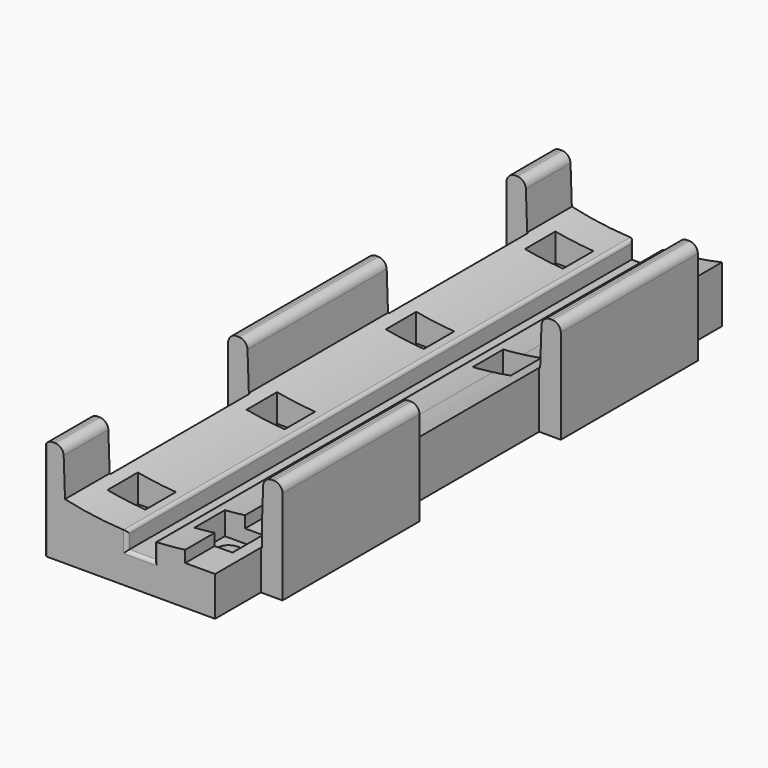
from build123d import *

# Parameters (mm, degrees)
F1_DEPTH     = 185
F3_DEPTH     = 30
F2_W         = 6.328
F2_H         = 51.6
F2_H_2       = 16.7
F2_H_3       = 50.8
F4_DEPTH     = 30
F5_D         = 6.7564
F6_START     = -7.6
F2_W_2       = 5.5565
F2_H_4       = 5.5565
F6_DEPTH     = 22.401
F7_T1_DEPTH  = 8
F7_T3_DEPTH  = 7.5701702527
F7_T5_DEPTH  = 35
F7_T7_DEPTH  = 189.78118177
F7_T13_DEPTH = 10.5
F7_T17_DEPTH = 10.0701702527
F7_T24_DEPTH = 10.0701702527
F7_T28_DEPTH = 10.5
F7_T35_DEPTH = 10.5
F7_T39_DEPTH = 10.0701702527
F7_T46_DEPTH = 10.0701702527
F7_T50_DEPTH = 10.5
F8_T1_DEPTH  = 27.8
F8_T3_DEPTH  = 28.3686226101
F8_T5_DEPTH  = 62.8686226101
F8_T7_DEPTH  = 63.3
F8_T9_DEPTH  = 27.8
F8_T11_DEPTH = 28.3686226101
F8_T13_DEPTH = 62.0686226101
F8_T15_DEPTH = 62.5
F8_T17_DEPTH = 62.5
F8_T19_DEPTH = 62.0686226101


# Not quite as in the source:
# - a fillet or chamfer that OpenCascade refuses, or shapes differently, is made with other operations: its cross-section is extruded or revolved along the edge and cut away or added
# - a feature names something its author has since deleted; it is built from what else it names


with BuildPart() as f1:
    # F0 (on Front) → F1 (new body)
    with BuildSketch(Plane.XZ):
        with BuildLine():
            Line((-28.0998, -84.153), (-28.0998, -96.0750292217))
            ThreePointArc((-28.0998, -96.0750292217), (-25.0871251247, -96.9053463591), (-22.05, -97.6412182431))
            Line((-22.05, -97.6412182431), (-22.5238, -84.153))
            Line((-22.5238, -84.153), (-28.0998, -84.153))
        make_face()
        with BuildLine():
            ThreePointArc((22.05, -97.6412182431), (25.0871251247, -96.9053463591), (28.0998, -96.0750292217))
            Line((28.0998, -96.0750292217), (28.0998, -84.153))
            Line((28.0998, -84.153), (22.5238, -84.153))
            Line((22.5238, -84.153), (22.05, -97.6412182431))
        make_face()
        with BuildLine():
            Line((22.05, -102.6412182431), (22.05, -97.6412182431))
            ThreePointArc((22.05, -97.6412182431), (17.5683261722, -98.5462526711), (13.05, -99.2456926017))
            Line((13.05, -99.2456926017), (13.05, -102.6412182431))
            Line((13.05, -102.6412182431), (22.05, -102.6412182431))
        make_face()
        with BuildLine():
            ThreePointArc((-22.05, -97.6412182431), (-25.0871251247, -96.9053463591), (-28.0998, -96.0750292217))
            Line((-28.0998, -96.0750292217), (-28.0998, -104.153))
            Line((-28.0998, -104.153), (-28.0998, -114.153))
            Line((-28.0998, -114.153), (0, -114.153))
            Line((0, -114.153), (28.0998, -114.153))
            Line((28.0998, -114.153), (28.0998, -104.153))
            Line((28.0998, -104.153), (28.0998, -96.0750292217))
            ThreePointArc((28.0998, -96.0750292217), (25.0871251247, -96.9053463591), (22.05, -97.6412182431))
            Line((22.05, -97.6412182431), (22.05, -102.6412182431))
            Line((22.05, -102.6412182431), (13.05, -102.6412182431))
            Line((13.05, -102.6412182431), (13.05, -99.2456926017))
            ThreePointArc((13.05, -99.2456926017), (8.5337876448, -99.7355727333), (4, -100.0200479904))
            Line((4, -100.0200479904), (4, -105.0902182431))
            Line((4, -105.0902182431), (-4, -105.0902182431))
            Line((-4, -105.0902182431), (-4, -100.0200479904))
            ThreePointArc((-4, -100.0200479904), (-13.0791946519, -99.2418493744), (-22.05, -97.6412182431))
        make_face()
    extrude(amount=-F1_DEPTH)

    # F0 (on Front) → F3 (cut)
    with BuildSketch(Plane.XZ):
        with BuildLine():
            Line((22.05, -102.6412182431), (22.05, -97.6412182431))
            ThreePointArc((22.05, -97.6412182431), (17.5683261722, -98.5462526711), (13.05, -99.2456926017))
            Line((13.05, -99.2456926017), (13.05, -102.6412182431))
            Line((13.05, -102.6412182431), (22.05, -102.6412182431))
        make_face()
    extrude(amount=-F3_DEPTH, mode=Mode.SUBTRACT)

    # F2 (on face) → F4 (cut, through all)
    with BuildSketch(Plane(origin=(0, 0, -114.153), x_dir=(1, 0, 0), z_dir=(0, 0, -1))):
        with Locations((24.9358, -92.5)):
            Rectangle(F2_W, F2_H)
        with Locations((24.9358, -176.65)):
            Rectangle(F2_W, F2_H_2)
        with Locations((24.9358, -8.35)):
            Rectangle(F2_W, F2_H_2)
        with Locations((-24.9358, -143.3)):
            Rectangle(F2_W, F2_H_3)
        with Locations((-24.9358, -41.7)):
            Rectangle(F2_W, F2_H_3)
    extrude(amount=-F4_DEPTH, mode=Mode.SUBTRACT)

    # F5 (through all)
    with Locations(Plane(origin=(0, 0, -114.153), x_dir=(1, 0, 0), z_dir=(0, 0, -1))):
        with Locations((-12.7, -168.7), (12.7, -168.7), (-12.7, -117.9), (12.7, -117.9), (-12.7, -67.1), (12.7, -67.1), (-12.7, -16.3), (12.7, -16.3)):
            Hole(F5_D / 2)

    # F2 (on face) → F6 (cut)
    with BuildSketch(Plane(origin=(0, 0, -114.153), x_dir=(1, 0, 0), z_dir=(0, 0, -1)).offset(F6_START)):
        Polygon((-12.7, -174.2565), (-12.7, -168.7), (-12.7, -163.1435), (-18.2565, -163.1435), (-18.2565, -174.2565), align=None)
        with Locations((-9.92175, -165.92175)):
            Rectangle(F2_W_2, F2_H_4)
        with Locations((-9.92175, -171.47825)):
            Rectangle(F2_W_2, F2_H_4)
        with Locations((9.92175, -171.47825)):
            Rectangle(F2_W_2, F2_H_4)
        with Locations((9.92175, -165.92175)):
            Rectangle(F2_W_2, F2_H_4)
        Polygon((12.7, -163.1435), (12.7, -168.7), (12.7, -174.2565), (18.2565, -174.2565), (18.2565, -163.1435), align=None)
        Polygon((12.7, -112.3435), (12.7, -117.9), (12.7, -123.4565), (18.2565, -123.4565), (18.2565, -112.3435), align=None)
        with Locations((9.92175, -115.12175)):
            Rectangle(F2_W_2, F2_H_4)
        with Locations((9.92175, -120.67825)):
            Rectangle(F2_W_2, F2_H_4)
        with Locations((-9.92175, -120.67825)):
            Rectangle(F2_W_2, F2_H_4)
        with Locations((-9.92175, -115.12175)):
            Rectangle(F2_W_2, F2_H_4)
        Polygon((-12.7, -123.4565), (-12.7, -117.9), (-12.7, -112.3435), (-18.2565, -112.3435), (-18.2565, -123.4565), align=None)
        with Locations((-9.92175, -64.32175)):
            Rectangle(F2_W_2, F2_H_4)
        with Locations((-9.92175, -69.87825)):
            Rectangle(F2_W_2, F2_H_4)
        Polygon((-12.7, -72.6565), (-12.7, -67.1), (-12.7, -61.5435), (-18.2565, -61.5435), (-18.2565, -72.6565), align=None)
        with Locations((9.92175, -64.32175)):
            Rectangle(F2_W_2, F2_H_4)
        with Locations((9.92175, -69.87825)):
            Rectangle(F2_W_2, F2_H_4)
        Polygon((12.7, -61.5435), (12.7, -67.1), (12.7, -72.6565), (18.2565, -72.6565), (18.2565, -61.5435), align=None)
        with Locations((9.92175, -19.07825)):
            Rectangle(F2_W_2, F2_H_4)
        with Locations((9.92175, -13.52175)):
            Rectangle(F2_W_2, F2_H_4)
        Polygon((18.2565, -10.7435), (12.7, -10.7435), (12.7, -16.3), (12.7, -21.8565), (18.2565, -21.8565), align=None)
        with Locations((-9.92175, -13.52175)):
            Rectangle(F2_W_2, F2_H_4)
        Polygon((-12.7, -16.3), (-12.7, -10.7435), (-18.2565, -10.7435), (-18.2565, -21.8565), (-12.7, -21.8565), align=None)
        with Locations((-9.92175, -19.07825)):
            Rectangle(F2_W_2, F2_H_4)
    extrude(amount=-F6_DEPTH, mode=Mode.SUBTRACT)

    # F7: fillet of radius 1 on 10 edges, made by hand

    # F7_s2 → F7_t1 (cut)
    with BuildSketch(Plane.YZ.offset(-4)):
        with BuildLine():
            ThreePointArc((0, -106.0902182431), (0.2928932188, -105.3831114619), (1, -105.0902182431))
            Line((1, -105.0902182431), (0, -105.0902182431))
            Line((0, -105.0902182431), (0, -106.0902182431))
        make_face()
        with BuildLine():
            ThreePointArc((184, -105.0902182431), (184.7071067812, -105.3831114619), (185, -106.0902182431))
            Line((185, -106.0902182431), (185, -105.0902182431))
            Line((185, -105.0902182431), (184, -105.0902182431))
        make_face()
    extrude(amount=F7_T1_DEPTH, mode=Mode.SUBTRACT)

    # F7_s4 → F7_t3 (cut)
    with BuildSketch(Plane.XY.offset(-105.0902182431)):
        with BuildLine():
            ThreePointArc((-5, 0), (-4.2928932188, 0.2928932188), (-4, 1))
            Line((-4, 1), (-4, 0))
            Line((-4, 0), (-5, 0))
        make_face()
        with BuildLine():
            ThreePointArc((5, 0), (4.2928932188, 0.2928932188), (4, 1))
            Line((4, 1), (4, 0))
            Line((4, 0), (5, 0))
        make_face()
        with BuildLine():
            ThreePointArc((-4, 184), (-4.2928932188, 184.7071067812), (-5, 185))
            Line((-5, 185), (-4, 185))
            Line((-4, 185), (-4, 184))
        make_face()
        with BuildLine():
            ThreePointArc((4, 184), (4.2928932188, 184.7071067812), (5, 185))
            Line((5, 185), (4, 185))
            Line((4, 185), (4, 184))
        make_face()
    extrude(amount=F7_T3_DEPTH, mode=Mode.SUBTRACT)

    # F7_s6 → F7_t5 (cut)
    with BuildSketch(Plane.XY.offset(-116.653)):
        with BuildLine():
            ThreePointArc((-27.0998, 0), (-27.8069067812, 0.2928932188), (-28.0998, 1))
            Line((-28.0998, 1), (-28.0998, 0))
            Line((-28.0998, 0), (-27.0998, 0))
        make_face()
        with BuildLine():
            ThreePointArc((-27.0998, 185), (-27.8069067812, 184.7071067812), (-28.0998, 184))
            Line((-28.0998, 184), (-28.0998, 185))
            Line((-28.0998, 185), (-27.0998, 185))
        make_face()
    extrude(amount=F7_T5_DEPTH, mode=Mode.SUBTRACT)

    # F7_s8 → F7_t7 (cut)
    with BuildSketch(Plane.XZ.offset(-187.390590885)):
        with BuildLine():
            ThreePointArc((-4.9505440158, -99.9775080403), (-4.2756188903, -100.2868845998), (-4, -100.9762843444))
            Line((-4, -100.9762843444), (-4, -100.0200479904))
            ThreePointArc((-4, -100.0200479904), (-4.4753225534, -99.9999074402), (-4.9505440158, -99.9775080403))
        make_face()
        with BuildLine():
            ThreePointArc((4, -100.9762843444), (4.2756188903, -100.2868845998), (4.9505440158, -99.9775080403))
            ThreePointArc((4.9505440158, -99.9775080403), (4.4753225534, -99.9999074402), (4, -100.0200479904))
            Line((4, -100.0200479904), (4, -100.9762843444))
        make_face()
    extrude(amount=F7_T7_DEPTH, mode=Mode.SUBTRACT)


with BuildPart() as f7_tool11:
    # F7_s12 → F7_t13 (new body)
    with BuildSketch(Plane.YZ.offset(6.5)):
        with BuildLine():
            ThreePointArc((0, -106.0902182431), (0.2928932188, -105.3831114619), (1, -105.0902182431))
            Line((1, -105.0902182431), (0, -105.0902182431))
            Line((0, -105.0902182431), (0, -106.0902182431))
        make_face()
    extrude(amount=-F7_T13_DEPTH)

    split(bisect_by=Plane.YZ.offset(4), keep=Keep.TOP)


with BuildPart() as f7_tool15:
    # F7_s16 → F7_t17 (new body)
    with BuildSketch(Plane.XY.offset(-97.5200479904)):
        with BuildLine():
            ThreePointArc((5, 0), (4.2928932188, 0.2928932188), (4, 1))
            Line((4, 1), (4, 0))
            Line((4, 0), (5, 0))
        make_face()
    extrude(amount=-F7_T17_DEPTH)

    split(bisect_by=Plane.XY.offset(-105.0902182431), keep=Keep.BOTTOM)


with BuildPart() as f7_tool11_1:
    add(f7_tool11.part)

    # F7_t19: intersect F7_tool15
    add(f7_tool15.part, mode=Mode.INTERSECT)


with BuildPart() as f1_1:
    add(f1.part)

    # F7_t9: cut F7_tool11
    add(f7_tool11_1.part, mode=Mode.SUBTRACT)


with BuildPart() as f7_tool22:
    # F7_s23 → F7_t24 (new body)
    with BuildSketch(Plane.XY.offset(-107.5902182431)):
        with BuildLine():
            ThreePointArc((-5, 0), (-4.2928932188, 0.2928932188), (-4, 1))
            Line((-4, 1), (-4, 0))
            Line((-4, 0), (-5, 0))
        make_face()
    extrude(amount=F7_T24_DEPTH)

    split(bisect_by=Plane.XY.offset(-105.0902182431), keep=Keep.BOTTOM)


with BuildPart() as f7_tool26:
    # F7_s27 → F7_t28 (new body)
    with BuildSketch(Plane.YZ.offset(4)):
        with BuildLine():
            ThreePointArc((0, -106.0902182431), (0.2928932188, -105.3831114619), (1, -105.0902182431))
            Line((1, -105.0902182431), (0, -105.0902182431))
            Line((0, -105.0902182431), (0, -106.0902182431))
        make_face()
    extrude(amount=-F7_T28_DEPTH)

    split(bisect_by=Plane.YZ.offset(-4), keep=Keep.BOTTOM)


with BuildPart() as f7_tool22_1:
    add(f7_tool22.part)

    # F7_t30: intersect F7_tool26
    add(f7_tool26.part, mode=Mode.INTERSECT)


with BuildPart() as f1_2:
    add(f1_1.part)

    # F7_t20: cut F7_tool22
    add(f7_tool22_1.part, mode=Mode.SUBTRACT)


with BuildPart() as f7_tool33:
    # F7_s34 → F7_t35 (new body)
    with BuildSketch(Plane.YZ.offset(6.5)):
        with BuildLine():
            ThreePointArc((184, -105.0902182431), (184.7071067812, -105.3831114619), (185, -106.0902182431))
            Line((185, -106.0902182431), (185, -105.0902182431))
            Line((185, -105.0902182431), (184, -105.0902182431))
        make_face()
    extrude(amount=-F7_T35_DEPTH)

    split(bisect_by=Plane.YZ.offset(4), keep=Keep.TOP)


with BuildPart() as f7_tool37:
    # F7_s38 → F7_t39 (new body)
    with BuildSketch(Plane.XY.offset(-97.5200479904)):
        with BuildLine():
            ThreePointArc((4, 184), (4.2928932188, 184.7071067812), (5, 185))
            Line((5, 185), (4, 185))
            Line((4, 185), (4, 184))
        make_face()
    extrude(amount=-F7_T39_DEPTH)

    split(bisect_by=Plane.XY.offset(-105.0902182431), keep=Keep.BOTTOM)


with BuildPart() as f7_tool33_1:
    add(f7_tool33.part)

    # F7_t41: intersect F7_tool37
    add(f7_tool37.part, mode=Mode.INTERSECT)


with BuildPart() as f1_3:
    add(f1_2.part)

    # F7_t31: cut F7_tool33
    add(f7_tool33_1.part, mode=Mode.SUBTRACT)


with BuildPart() as f7_tool44:
    # F7_s45 → F7_t46 (new body)
    with BuildSketch(Plane.XY.offset(-107.5902182431)):
        with BuildLine():
            ThreePointArc((-4, 184), (-4.2928932188, 184.7071067812), (-5, 185))
            Line((-5, 185), (-4, 185))
            Line((-4, 185), (-4, 184))
        make_face()
    extrude(amount=F7_T46_DEPTH)

    split(bisect_by=Plane.XY.offset(-105.0902182431), keep=Keep.BOTTOM)


with BuildPart() as f7_tool48:
    # F7_s49 → F7_t50 (new body)
    with BuildSketch(Plane.YZ.offset(4)):
        with BuildLine():
            ThreePointArc((184, -105.0902182431), (184.7071067812, -105.3831114619), (185, -106.0902182431))
            Line((185, -106.0902182431), (185, -105.0902182431))
            Line((185, -105.0902182431), (184, -105.0902182431))
        make_face()
    extrude(amount=-F7_T50_DEPTH)

    split(bisect_by=Plane.YZ.offset(-4), keep=Keep.BOTTOM)


with BuildPart() as f7_tool44_1:
    add(f7_tool44.part)

    # F7_t52: intersect F7_tool48
    add(f7_tool48.part, mode=Mode.INTERSECT)


with BuildPart() as f1_4:
    add(f1_3.part)

    # F7_t42: cut F7_tool44
    add(f7_tool44_1.part, mode=Mode.SUBTRACT)

    # F8: fillet of radius 2.5 on 10 edges, made by hand

    # F8_s2 → F8_t1 (cut)
    with BuildSketch(Plane.XZ.offset(-22.55)):
        with BuildLine():
            ThreePointArc((-28.0998, -86.653), (-27.367566953, -84.885233047), (-25.5998, -84.153))
            Line((-25.5998, -84.153), (-28.0998, -84.153))
            Line((-28.0998, -84.153), (-28.0998, -86.653))
        make_face()
    extrude(amount=F8_T1_DEPTH, mode=Mode.SUBTRACT)

    # F8_s4 → F8_t3 (cut)
    with BuildSketch(Plane.XZ.offset(-22.3343113051)):
        with BuildLine():
            ThreePointArc((-22.4390654746, -86.565236748), (-23.2010637724, -84.8544716947), (-24.937524522, -84.153))
            Line((-24.937524522, -84.153), (-22.5238, -84.153))
            Line((-22.5238, -84.153), (-22.4390654746, -86.565236748))
        make_face()
    extrude(amount=F8_T3_DEPTH, mode=Mode.SUBTRACT)

    # F8_s6 → F8_t5 (cut)
    with BuildSketch(Plane.XZ.offset(-123.9343113051)):
        with BuildLine():
            ThreePointArc((-24.937524522, -84.153), (-23.2010637724, -84.8544716947), (-22.4390654746, -86.565236748))
            Line((-22.4390654746, -86.565236748), (-22.5238, -84.153))
            Line((-22.5238, -84.153), (-24.937524522, -84.153))
        make_face()
    extrude(amount=F8_T5_DEPTH, mode=Mode.SUBTRACT)

    # F8_s8 → F8_t7 (cut)
    with BuildSketch(Plane.XZ.offset(-124.15)):
        with BuildLine():
            ThreePointArc((-28.0998, -86.653), (-27.367566953, -84.885233047), (-25.5998, -84.153))
            Line((-25.5998, -84.153), (-28.0998, -84.153))
            Line((-28.0998, -84.153), (-28.0998, -86.653))
        make_face()
    extrude(amount=F8_T7_DEPTH, mode=Mode.SUBTRACT)

    # F8_s10 → F8_t9 (cut)
    with BuildSketch(Plane.XZ.offset(-190.25)):
        with BuildLine():
            ThreePointArc((-28.0998, -86.653), (-27.367566953, -84.885233047), (-25.5998, -84.153))
            Line((-25.5998, -84.153), (-28.0998, -84.153))
            Line((-28.0998, -84.153), (-28.0998, -86.653))
        make_face()
    extrude(amount=F8_T9_DEPTH, mode=Mode.SUBTRACT)

    # F8_s12 → F8_t11 (cut)
    with BuildSketch(Plane.XZ.offset(-191.0343113051)):
        with BuildLine():
            ThreePointArc((-24.937524522, -84.153), (-23.2010637724, -84.8544716947), (-22.4390654746, -86.565236748))
            Line((-22.4390654746, -86.565236748), (-22.5238, -84.153))
            Line((-22.5238, -84.153), (-24.937524522, -84.153))
        make_face()
    extrude(amount=F8_T11_DEPTH, mode=Mode.SUBTRACT)

    # F8_s14 → F8_t13 (cut)
    with BuildSketch(Plane.XZ.offset(-174.3343113051)):
        with BuildLine():
            ThreePointArc((22.4390654746, -86.565236748), (23.2010637724, -84.8544716947), (24.937524522, -84.153))
            Line((24.937524522, -84.153), (22.5238, -84.153))
            Line((22.5238, -84.153), (22.4390654746, -86.565236748))
        make_face()
    extrude(amount=F8_T13_DEPTH, mode=Mode.SUBTRACT)

    # F8_s16 → F8_t15 (cut)
    with BuildSketch(Plane.XZ.offset(-174.55)):
        with BuildLine():
            ThreePointArc((25.5998, -84.153), (27.367566953, -84.885233047), (28.0998, -86.653))
            Line((28.0998, -86.653), (28.0998, -84.153))
            Line((28.0998, -84.153), (25.5998, -84.153))
        make_face()
    extrude(amount=F8_T15_DEPTH, mode=Mode.SUBTRACT)

    # F8_s18 → F8_t17 (cut)
    with BuildSketch(Plane.XZ.offset(-72.95)):
        with BuildLine():
            ThreePointArc((25.5998, -84.153), (27.367566953, -84.885233047), (28.0998, -86.653))
            Line((28.0998, -86.653), (28.0998, -84.153))
            Line((28.0998, -84.153), (25.5998, -84.153))
        make_face()
    extrude(amount=F8_T17_DEPTH, mode=Mode.SUBTRACT)

    # F8_s20 → F8_t19 (cut)
    with BuildSketch(Plane.XZ.offset(-72.7343113051)):
        with BuildLine():
            ThreePointArc((22.4390654746, -86.565236748), (23.2010637724, -84.8544716947), (24.937524522, -84.153))
            Line((24.937524522, -84.153), (22.5238, -84.153))
            Line((22.5238, -84.153), (22.4390654746, -86.565236748))
        make_face()
    extrude(amount=F8_T19_DEPTH, mode=Mode.SUBTRACT)


solid = f1_4.part
